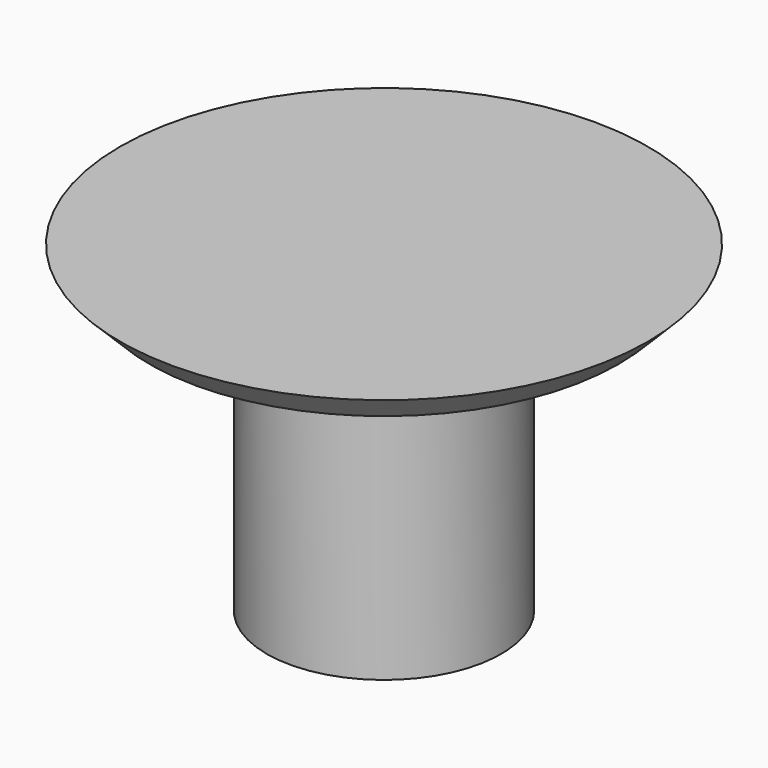
from build123d import *

# Parameters (mm, degrees)
F0_W   = 4
F0_H   = 1
F0_W_2 = 1.5
F0_H_2 = 0.5


# Not quite as in the source:
# - a fillet or chamfer that OpenCascade refuses, or shapes differently, is made with other operations: its cross-section is extruded or revolved along the edge and cut away or added


with BuildPart() as f1:
    # F0 (on Front) → F1 (revolve)
    with BuildSketch(Plane.XZ):
        with Locations((-2, -0.5)):
            Rectangle(F0_W, F0_H)
        Polygon((-4, 0), (0, 0), (0, 10), (-4, 10), (-4, 9), (-4, 8.5), align=None)
        with Locations((-4.75, 8.75)):
            Rectangle(F0_W_2, F0_H_2)
        Polygon((-4, 9), (-4, 10), (-11, 10), (-11, 9), (-5.5, 9), align=None)
    revolve(axis=Axis((0, 0, 5), (0, 0, 1)))

    # F2: chamfer of 3 on 1 edges, made by hand

    # F2_s1 → F2_t2 (revolve, cut)
    with BuildSketch(Plane.XZ):
        Polygon((-11, 12), (-8, 9), (-11, 9), align=None)
    revolve(axis=Axis((0, 0, 9), (0, 0, 1)), mode=Mode.SUBTRACT)


solid = f1.part
